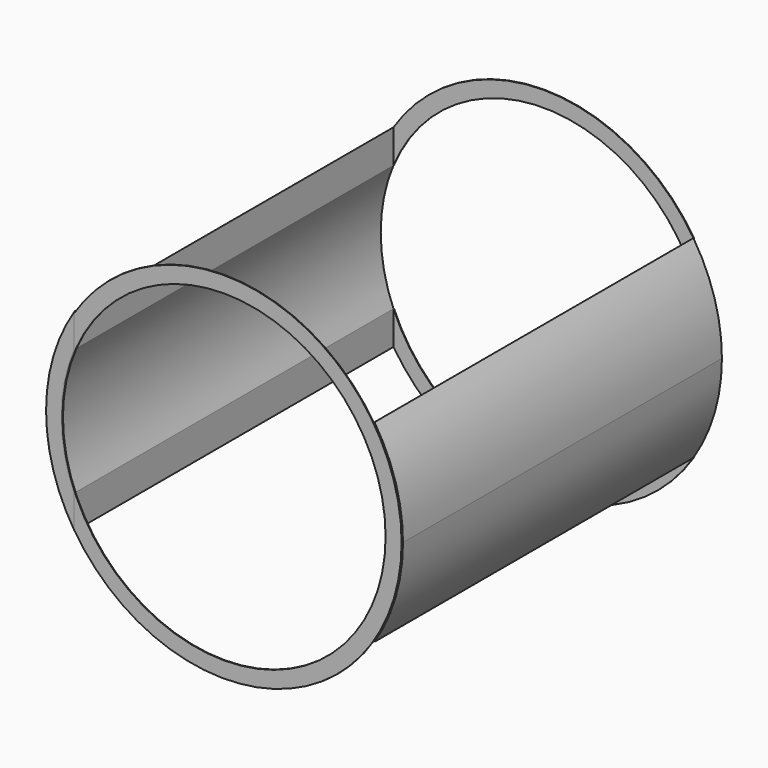
from build123d import *

# Parameters (mm, degrees)
F1_DEPTH = 303.8
F2_DEPTH = 0.5
F3_R     = 123.138814649
F4_DEPTH = 0.508


# Not quite as in the source:
# - ends of sketch curves that miss each other by under 0.0002 mm in the source are joined


with BuildPart() as f1:
    # F0 (on Front) → F1 (new body)
    with BuildSketch(Plane.XZ):
        with BuildLine():
            Line((-236.8527790219, -113.4836752775), (-236.8527790219, -87.8702830895))
            ThreePointArc((-236.8527790219, -87.8702830895), (-258.5527790219, -161.5690619125), (-236.8527790219, -235.2678407355))
            Line((-236.8527790219, -235.2678407355), (-236.8527790219, -209.6544485476))
            ThreePointArc((-236.8527790219, -209.6544485476), (-246.5555790219, -161.5690619125), (-236.8527790219, -113.4836752775))
        make_face()
    extrude(amount=F1_DEPTH)



with BuildPart() as f1b:
    # F0 (on Front) → F1, piece 2 (new body)
    with BuildSketch(Plane.XZ):
        with BuildLine():
            ThreePointArc((-8.2527790219, -235.2678407355), (7.909476056, -199.9826011923), (13.4472209781, -161.5690619125))
            ThreePointArc((13.4472209781, -161.5690619125), (7.909476056, -123.1555226327), (-8.2527790219, -87.8702830895))
            Line((-8.2527790219, -87.8702830895), (-8.2527790219, -113.4836752775))
            ThreePointArc((-8.2527790219, -113.4836752775), (-0.999880151, -137.0417876261), (1.4500209781, -161.5690619125))
            ThreePointArc((1.4500209781, -161.5690619125), (-0.999880151, -186.0963361989), (-8.2527790219, -209.6544485476))
            Line((-8.2527790219, -209.6544485476), (-8.2527790219, -235.2678407355))
        make_face()
    extrude(amount=F1_DEPTH)


with BuildPart() as f2:
    # F0 (on Front) → F2 (new body)
    with BuildSketch(Plane.XZ):
        with BuildLine():
            Line((-8.2527790219, -113.4836752775), (-8.2527790219, -87.8702830895))
            ThreePointArc((-8.2527790219, -87.8702830895), (-122.5528719649, -25.5690619126), (-236.8527790219, -87.8702830895))
            Line((-236.8527790219, -87.8702830895), (-236.8527790219, -113.4836752775))
            ThreePointArc((-236.8527790219, -113.4836752775), (-122.5527790219, -37.5662619125), (-8.2527790219, -113.4836752775))
        make_face()
    extrude(amount=-F2_DEPTH)


with BuildPart() as f2b:
    # F0 (on Front) → F2, piece 2 (new body)
    with BuildSketch(Plane.XZ):
        with BuildLine():
            ThreePointArc((-236.8527790219, -235.2678407355), (-122.5527790219, -297.5690619125), (-8.2527790219, -235.2678407355))
            Line((-8.2527790219, -235.2678407355), (-8.2527790219, -209.6544485476))
            ThreePointArc((-8.2527790219, -209.6544485476), (-122.5527790219, -285.5718619125), (-236.8527790219, -209.6544485476))
            Line((-236.8527790219, -209.6544485476), (-236.8527790219, -235.2678407355))
        make_face()
    extrude(amount=-F2_DEPTH)


with BuildPart() as f1_1:
    add(f1.part)

    add(f1b.part)  # F4 merges F1b
    # F3 (on face) → F4 (join)
    with BuildSketch(Plane.XZ.offset(303.8)):
        with BuildLine():
            ThreePointArc((-236.8527790219, -234.0665643946), (-84.8065611673, -291.5521412106), (12.8000113673, -161.5690619125))
            ThreePointArc((12.8000113673, -161.5690619125), (-84.8065611673, -31.5859826145), (-236.8527790219, -89.0715594305))
            Line((-236.8527790219, -89.0715594305), (-236.8527790219, -113.4836752775))
            ThreePointArc((-236.8527790219, -113.4836752775), (-246.5555790219, -161.5690619125), (-236.8527790219, -209.6544485476))
            Line((-236.8527790219, -209.6544485476), (-236.8527790219, -234.0665643946))
        make_face()
        with Locations((-122.5527790219, -161.5690619125)):
            Circle(F3_R, mode=Mode.SUBTRACT)
    extrude(amount=F4_DEPTH)


solid = Compound([f2.part, f2b.part, f1_1.part])
